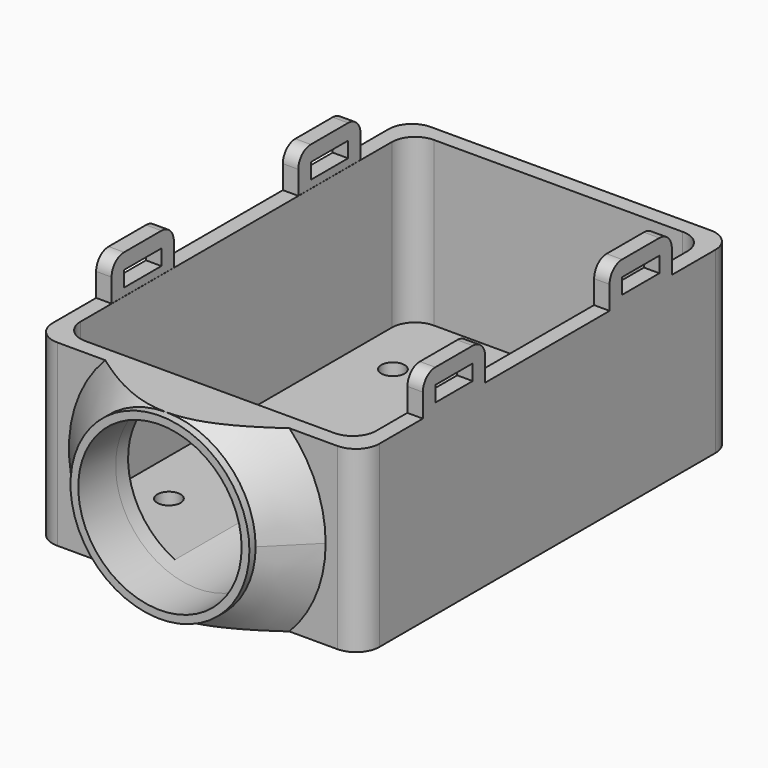
from build123d import *

# Parameters (mm, degrees)
F4_DEPTH     = 23
F5_DEPTH     = 2
F6_R         = 11.5
F6_R_2       = 10.5
F7_DEPTH     = 6
F8_DEPTH     = 25
F9_T4_ANGLE  = 179.9999999711
F9_T10_ANGLE = 89.9999998967
F9_T15_ANGLE = 90.0000001322
F10_R        = 1.5
F11_DEPTH    = 2.001
F12_W        = 1.9858112633
F12_H        = 10
F13_DEPTH    = 5
F14_R        = 2
F15_W        = 6
F15_H        = 2
F16_DEPTH    = 42.001


# Not quite as in the source:
# - a fillet or chamfer that OpenCascade refuses, or shapes differently, is made with other operations: its cross-section is extruded or revolved along the edge and cut away or added


with BuildPart() as f4:
    # F3 (on Top) → F4 (new body)
    with BuildSketch(Plane.XY):
        with BuildLine():
            Line((18, 30), (-18, 30))
            ThreePointArc((-18, 30), (-20.1213203436, 29.1213203436), (-21, 27))
            Line((-21, 27), (-21, -27))
            ThreePointArc((-21, -27), (-20.1213203436, -29.1213203436), (-18, -30))
            Line((-18, -30), (18, -30))
            ThreePointArc((18, -30), (20.1213203436, -29.1213203436), (21, -27))
            Line((21, -27), (21, 27))
            ThreePointArc((21, 27), (20.1213203436, 29.1213203436), (18, 30))
        make_face()
        with BuildLine():
            ThreePointArc((-19, 25), (-18.1213203436, 27.1213203436), (-16, 28))
            Line((-16, 28), (16, 28))
            ThreePointArc((16, 28), (18.1213203436, 27.1213203436), (19, 25))
            Line((19, 25), (19, -25))
            ThreePointArc((19, -25), (18.1213203436, -27.1213203436), (16, -28))
            Line((16, -28), (-16, -28))
            ThreePointArc((-16, -28), (-18.1213203436, -27.1213203436), (-19, -25))
            Line((-19, -25), (-19, 25))
        make_face(mode=Mode.SUBTRACT)
    extrude(amount=F4_DEPTH)

    # F3 (on Top) → F5 (join)
    with BuildSketch(Plane.XY):
        with BuildLine():
            Line((16, 28), (-16, 28))
            ThreePointArc((-16, 28), (-18.1213203436, 27.1213203436), (-19, 25))
            Line((-19, 25), (-19, -25))
            ThreePointArc((-19, -25), (-18.1213203436, -27.1213203436), (-16, -28))
            Line((-16, -28), (16, -28))
            ThreePointArc((16, -28), (18.1213203436, -27.1213203436), (19, -25))
            Line((19, -25), (19, 25))
            ThreePointArc((19, 25), (18.1213203436, 27.1213203436), (16, 28))
        make_face()
    extrude(amount=F5_DEPTH)

    # F6 (on face) → F7 (join)
    with BuildSketch(Plane.XZ.offset(30)):
        with Locations((0, 11.5)):
            Circle(F6_R)
        with Locations((0, 11.5)):
            Circle(F6_R_2, mode=Mode.SUBTRACT)
    extrude(amount=F7_DEPTH)

    # F8 (cut): a face of the model
    f8_faces = [f4.faces().sort_by_distance(p)[0] for p in [
        (0, -30, 11.5),
    ]]
    extrude(f8_faces, amount=-F8_DEPTH, mode=Mode.SUBTRACT)

    # F9: chamfer of 5 on 1 edges, made by hand


with BuildPart() as f9_tool2:
    # F9_s3 → F9_t4 (revolve)
    with BuildSketch(Plane.YZ):
        Polygon((-30, 28), (-35, 23), (-30, 23), align=None)
    revolve(axis=Axis((0, -30, 11.5), (0, -1, 0)), revolution_arc=F9_T4_ANGLE)

    split(bisect_by=Plane.XY, keep=Keep.TOP)

    split(bisect_by=Plane.XY.offset(23), keep=Keep.BOTTOM)


with BuildPart() as f4_1:
    add(f4.part)

    # F9_t1: union F9_tool2
    add(f9_tool2.part)


with BuildPart() as f9_tool8:
    # F9_s9 → F9_t10 (revolve)
    with BuildSketch(Plane.XY.offset(11.5)):
        Polygon((16.5, -30), (11.5, -35), (11.5, -30), align=None)
    revolve(axis=Axis((0, -30, 11.5), (0, -1, 0)), revolution_arc=F9_T10_ANGLE)

    split(bisect_by=Plane.XY.offset(23), keep=Keep.BOTTOM)


with BuildPart() as f4_2:
    add(f4_1.part)

    # F9_t7: union F9_tool8
    add(f9_tool8.part)


with BuildPart() as f9_tool13:
    # F9_s14 → F9_t15 (revolve)
    with BuildSketch(Plane.YZ):
        Polygon((-30, -5), (-35, 0), (-30, 0), align=None)
    revolve(axis=Axis((0, -30, 11.5), (0, -1, 0)), revolution_arc=F9_T15_ANGLE)

    split(bisect_by=Plane.XY, keep=Keep.TOP)


with BuildPart() as f4_3:
    add(f4_2.part)

    # F9_t12: union F9_tool13
    add(f9_tool13.part)

    # F10 (on face) → F11 (cut, through all)
    with BuildSketch(Plane.XY.offset(2)):
        with Locations((-13.25, 18)):
            Circle(F10_R)
        with Locations((-13.25, -18)):
            Circle(F10_R)
        with Locations((13.25, 18)):
            Circle(F10_R)
        with Locations((13.25, -18)):
            Circle(F10_R)
    extrude(amount=-F11_DEPTH, mode=Mode.SUBTRACT)

    # F12 (on face) → F13 (join)
    with BuildSketch(Plane.XY.offset(23)):
        with Locations((-20.0070943683, 15)):
            Rectangle(F12_W, F12_H)
        with Locations((-20.0070943683, -15)):
            Rectangle(F12_W, F12_H)
        with Locations((20.0070943683, 15)):
            Rectangle(F12_W, F12_H)
        with Locations((20.0070943683, -15)):
            Rectangle(F12_W, F12_H)
    extrude(amount=F13_DEPTH)

    # F14
    f14_edges = [f4_3.edges().sort_by_distance(p)[0] for p in [
        (-20.007094, -20, 28),
        (-20.007094, -10, 28),
        (-20.007094, 10, 28),
        (-20.007094, 20, 28),
        (20.007094, 20, 28),
        (20.007094, 10, 28),
        (20.007094, -10, 28),
        (20.007094, -20, 28),
    ]]
    fillet(f14_edges, radius=F14_R)

    # F15 (on face) → F16 (cut, through all)
    with BuildSketch(Plane(origin=(-21, 0, 0), x_dir=(0, -1, 0), z_dir=(-1, 0, 0))):
        with Locations((-15, 25)):
            Rectangle(F15_W, F15_H)
        with Locations((15, 25)):
            Rectangle(F15_W, F15_H)
    extrude(amount=-F16_DEPTH, mode=Mode.SUBTRACT)


solid = f4_3.part
